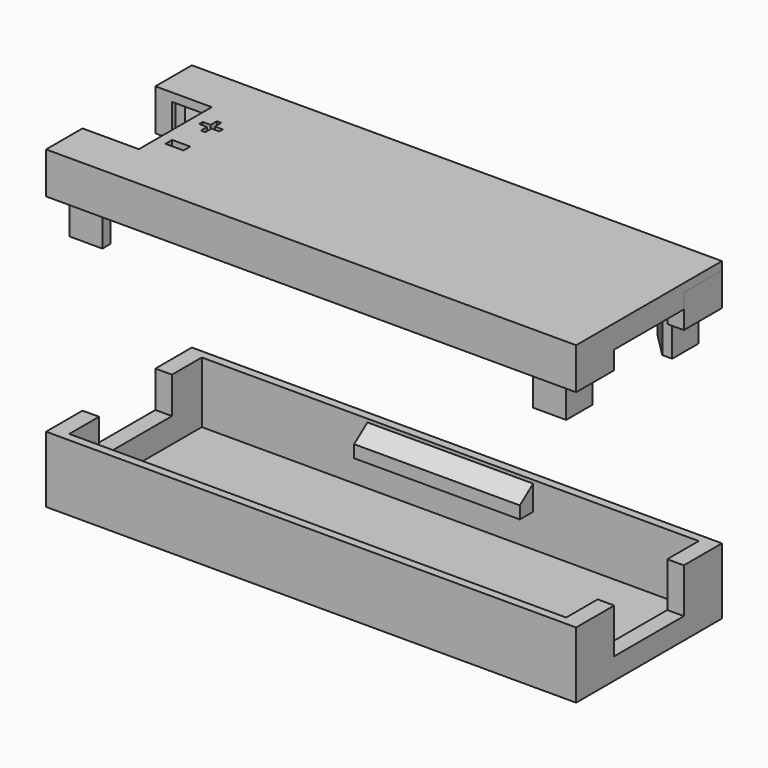
from build123d import *

# Parameters (mm, degrees)
F0_W            = 60
F0_H            = 20
F1_DEPTH        = 0.6
F0_W_2          = 64
F0_H_2          = 22
F2_DEPTH        = 8
F6_DEPTH        = 10
F7_W            = 10.5
F7_H            = 5.4
F8_DEPTH        = 2
F9_W            = 11
F9_H            = 4.4
F10_DEPTH       = 2
F12_W           = 2
F12_H           = 11
F12_W_2         = 2.0000000003
F12_H_2         = 10.5
F13_DEPTH       = 4
F14_W           = 64
F14_H           = 22
F15_DEPTH       = 1
F16_DEPTH       = 2.2
F17_W           = 6.8
F17_H           = 11
F18_DEPTH       = 5.001
F19_W           = 4
F19_H           = 4
F20_DEPTH       = 8
F21_SIZE        = 2.8
F22_TEXT_SIZE   = 5.0180156429
F22_TEXT_SIZE_2 = 8.3333333333
F23_DEPTH       = 1


# Not quite as in the source:
# - Text() gives the source's letters only with a copy of the font that has no kerning and outlines rounded to 1/6400 em; it was checked with that copy


with BuildPart() as f1:
    # F0 (on Top) → F1 (new body)
    with BuildSketch(Plane.XY):
        with Locations((-30, 10)):
            Rectangle(F0_W, F0_H)
    extrude(amount=F1_DEPTH)

    # F0 (on Top) → F2 (join)
    with BuildSketch(Plane.XY):
        with Locations((-30, 10)):
            Rectangle(F0_W_2, F0_H_2)
        with Locations((-30, 10)):
            Rectangle(F0_W, F0_H, mode=Mode.SUBTRACT)
    extrude(amount=F2_DEPTH)

    # F5 (on plane+point) → F6 (join, symmetric)
    with BuildSketch(Plane.YZ.offset(-30)):
        Polygon((2, 6.1), (0, 7.6), (0, 4.6), (2, 4.6), align=None)
        Polygon((20, 4.6), (20, 7.6), (18, 6.1), (18, 4.6), align=None)
    extrude(amount=F6_DEPTH, both=True)

    # F7 (on face) → F8 (cut, through all)
    with BuildSketch(Plane.YZ.offset(2)):
        with Locations((10, 5.3)):
            Rectangle(F7_W, F7_H)
    extrude(amount=-F8_DEPTH, mode=Mode.SUBTRACT)

    # F9 (on face) → F10 (cut, through all)
    with BuildSketch(Plane(origin=(-62, 0, 0), x_dir=(0, -1, 0), z_dir=(-1, 0, 0))):
        with Locations((-10, 5.8)):
            Rectangle(F9_W, F9_H)
    extrude(amount=-F10_DEPTH, mode=Mode.SUBTRACT)


with BuildPart() as f13:
    # F12 (on offset) → F13 (new body)
    with BuildSketch(Plane.XY.offset(33)):
        Polygon((-62, 21), (-62, 15.5), (-60, 15.5), (-60, 20), (0, 20), (0, 15.25), (1.9999999999, 15.25), (2, 21), align=None)
        with Locations((-61, 10)):
            Rectangle(F12_W, F12_H)
        Polygon((-60, 4.5), (-62, 4.5), (-62, -1), (2, -1), (2, 4.75), (-3e-10, 4.75), (0, 0), (-60, 0), align=None)
        with Locations((0.9999999998, 10)):
            Rectangle(F12_W_2, F12_H_2)
    extrude(amount=F13_DEPTH)

    # F14 (on face) → F15 (join)
    with BuildSketch(Plane.XY.offset(37)):
        with Locations((-30, 10)):
            Rectangle(F14_W, F14_H)
    extrude(amount=F15_DEPTH)

    # F12 (on offset) → F16 (cut)
    with BuildSketch(Plane.XY.offset(33)):
        with Locations((0.9999999998, 10)):
            Rectangle(F12_W_2, F12_H_2)
    extrude(amount=F16_DEPTH, mode=Mode.SUBTRACT)

    # F17 (on face) → F18 (cut, through all)
    with BuildSketch(Plane.XY.offset(38)):
        with Locations((-58.6, 10)):
            Rectangle(F17_W, F17_H)
    extrude(amount=-F18_DEPTH, mode=Mode.SUBTRACT)

    # F19 (on face) → F20 (join)
    with BuildSketch(Plane(origin=(0, 0, 37), x_dir=(1, 0, 0), z_dir=(0, 0, -1))):
        with Locations((-2, -18)):
            Rectangle(F19_W, F19_H)
        with Locations((-2, -2)):
            Rectangle(F19_W, F19_H)
        with Locations((-58, -2)):
            Rectangle(F19_W, F19_H)
        with Locations((-58, -18)):
            Rectangle(F19_W, F19_H)
    extrude(amount=F20_DEPTH)

    # F21
    f21_edges = [f13.edges().sort_by_distance(p)[0] for p in [
        (-56, 4, 33),
        (-56, 16, 33),
        (-4, 4, 33),
        (-4, 16, 33),
    ]]
    chamfer(f21_edges, length=F21_SIZE)

    # F22 (on face) → F23 (cut, through all)
    with BuildSketch(Plane.XY.offset(38)):
        with Locations((-54.1834567551, 10.5649182668)):
            Text('+', F22_TEXT_SIZE, font='Open Sans', font_style=FontStyle.BOLD, text_align=(TextAlign.LEFT, TextAlign.BOTTOM))
        with Locations((-54.1834567551, 5.2004032672)):
            Text('-', F22_TEXT_SIZE_2, font='Open Sans', font_style=FontStyle.BOLD, text_align=(TextAlign.LEFT, TextAlign.BOTTOM))
    extrude(amount=-F23_DEPTH, mode=Mode.SUBTRACT)


solid = Compound([f1.part, f13.part])
